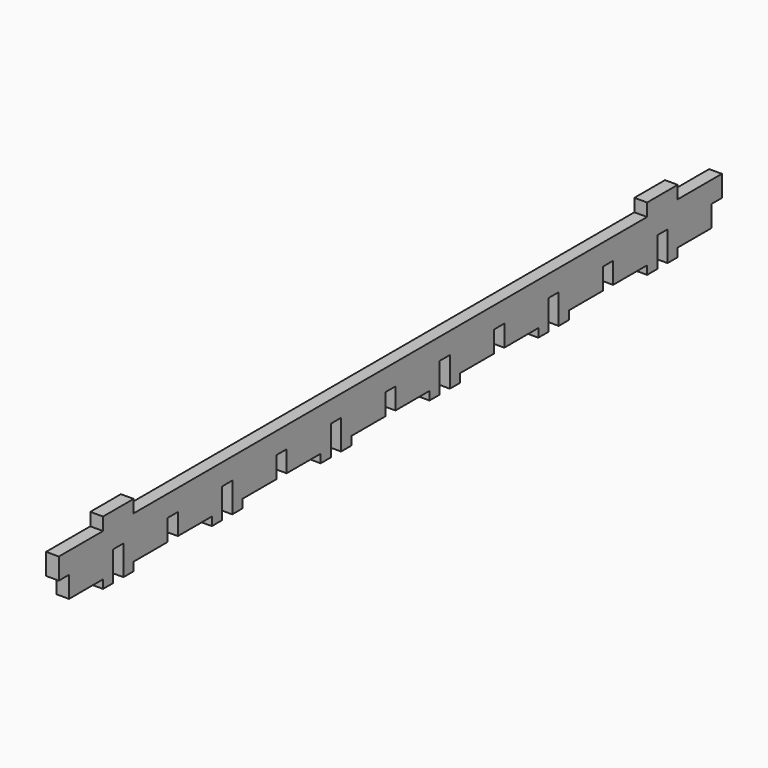
from build123d import *

# Parameters (mm, degrees)
F0_W     = 1.5
F0_H     = 5
F0_W_2   = 3
F0_H_2   = 2
F0_H_3   = 3
F1_DEPTH = 3


# Not quite as in the source:
# - a feature names something its author has since deleted; it is built from what else it names


with BuildPart() as f1:
    # F0 (on Right) → F1 (new body)
    with BuildSketch(Plane.YZ):
        Polygon((1.5, 5), (1.5, 0), (11.5, 0), (14.5, 0), (14.5, 5), (14.5, 10), (11.5, 10), (1.5, 10), align=None)
        with Locations((-0.75, 7.5)):
            Rectangle(F0_W, F0_H)
        with Locations((0.75, 7.5)):
            Rectangle(F0_W, F0_H)
        with Locations((13, -1)):
            Rectangle(F0_W_2, F0_H_2)
        with Locations((16, 7.5)):
            Rectangle(F0_W_2, F0_H)
        with Locations((19, -1)):
            Rectangle(F0_W_2, F0_H_2)
        Polygon((17.5, 5), (17.5, 0), (20.5, 0), (30.5, 0), (30.5, 5), (30.5, 10), (20.5, 10), (17.5, 10), align=None)
        with Locations((13, 11.5)):
            Rectangle(F0_W_2, F0_H_3)
        with Locations((16, 11.5)):
            Rectangle(F0_W_2, F0_H_3)
        with Locations((19, 11.5)):
            Rectangle(F0_W_2, F0_H_3)
        Polygon((33.5, 5), (33.5, 0), (43.5, 0), (46.5, 0), (46.5, 5), (46.5, 10), (33.5, 10), align=None)
        with Locations((32, 7.5)):
            Rectangle(F0_W_2, F0_H)
        with Locations((45, -1)):
            Rectangle(F0_W_2, F0_H_2)
        with Locations((48, 7.5)):
            Rectangle(F0_W_2, F0_H)
        with Locations((51, -1)):
            Rectangle(F0_W_2, F0_H_2)
        Polygon((49.5, 5), (49.5, 0), (52.5, 0), (62.5, 0), (62.5, 5), (62.5, 10), (49.5, 10), align=None)
        with Locations((64, 7.5)):
            Rectangle(F0_W_2, F0_H)
        Polygon((78.5, 10), (65.5, 10), (65.5, 5), (65.5, 0), (75.5, 0), (78.5, 0), (78.5, 5), align=None)
        with Locations((80, 7.5)):
            Rectangle(F0_W_2, F0_H)
        with Locations((77, -1)):
            Rectangle(F0_W_2, F0_H_2)
        Polygon((94.5, 10), (81.5, 10), (81.5, 5), (81.5, 0), (84.5, 0), (94.5, 0), (94.5, 5), align=None)
        with Locations((95.25, 7.5)):
            Rectangle(F0_W, F0_H)
        with Locations((83, -1)):
            Rectangle(F0_W_2, F0_H_2)
        with Locations((96.75, 7.5)):
            Rectangle(F0_W, F0_H)
        Polygon((110.5, 10), (97.5, 10), (97.5, 5), (97.5, 0), (107.5, 0), (110.5, 0), (110.5, 5), align=None)
        with Locations((112, 7.5)):
            Rectangle(F0_W_2, F0_H)
        Polygon((126.5, 10), (113.5, 10), (113.5, 5), (113.5, 0), (116.5, 0), (126.5, 0), (126.5, 5), align=None)
        with Locations((109, -1)):
            Rectangle(F0_W_2, F0_H_2)
        with Locations((128, 7.5)):
            Rectangle(F0_W_2, F0_H)
        with Locations((115, -1)):
            Rectangle(F0_W_2, F0_H_2)
        Polygon((142.5, 10), (129.5, 10), (129.5, 5), (129.5, 0), (139.5, 0), (142.5, 0), (142.5, 5), align=None)
        with Locations((144, 7.5)):
            Rectangle(F0_W_2, F0_H)
        Polygon((158.5, 10), (145.5, 10), (145.5, 5), (145.5, 0), (148.5, 0), (158.5, 0), (158.5, 5), align=None)
        with Locations((160, 7.5)):
            Rectangle(F0_W_2, F0_H)
        with Locations((141, -1)):
            Rectangle(F0_W_2, F0_H_2)
        with Locations((147, -1)):
            Rectangle(F0_W_2, F0_H_2)
        Polygon((171.5, 10), (161.5, 10), (161.5, 5), (161.5, 0), (171.5, 0), (174.5, 0), (174.5, 5), (174.5, 10), align=None)
        with Locations((173, 11.5)):
            Rectangle(F0_W_2, F0_H_3)
        with Locations((176, 11.5)):
            Rectangle(F0_W_2, F0_H_3)
        with Locations((176, 7.5)):
            Rectangle(F0_W_2, F0_H)
        with Locations((173, -1)):
            Rectangle(F0_W_2, F0_H_2)
        Polygon((180.5, 10), (177.5, 10), (177.5, 5), (177.5, 0), (180.5, 0), (190.5, 0), (190.5, 5), (190.5, 10), align=None)
        with Locations((179, 11.5)):
            Rectangle(F0_W_2, F0_H_3)
        with Locations((179, -1)):
            Rectangle(F0_W_2, F0_H_2)
        with Locations((191.25, 7.5)):
            Rectangle(F0_W, F0_H)
        with Locations((192.75, 7.5)):
            Rectangle(F0_W, F0_H)
    extrude(amount=F1_DEPTH)


solid = f1.part
